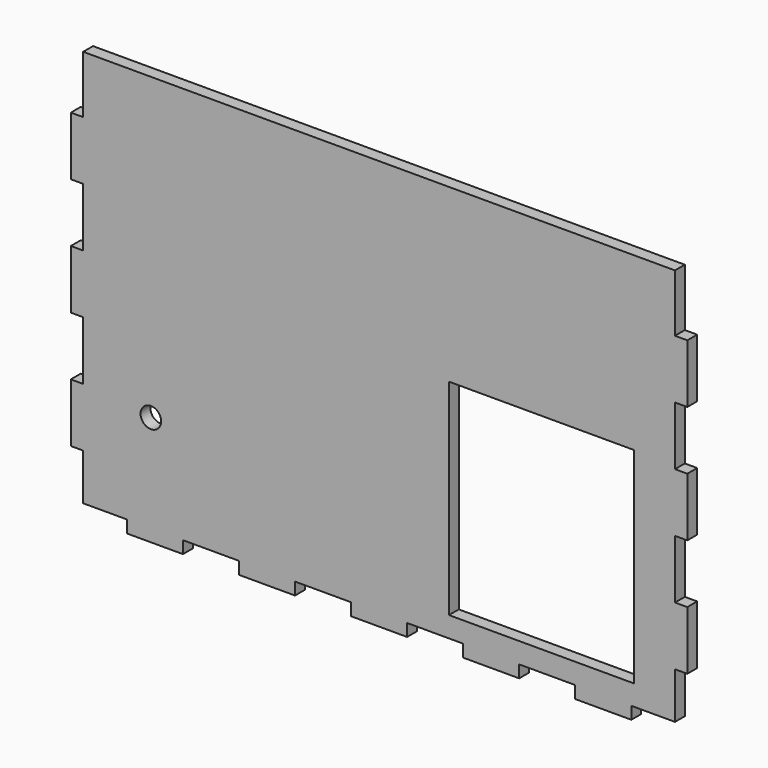
from build123d import *

# Parameters (mm, degrees)
F0_R     = 2.5
F0_W     = 45
F0_H     = 50
F1_DEPTH = 3


# Not quite as in the source:
# - ends of sketch curves that miss each other by under 0.0002 mm in the source are joined


with BuildPart() as f1:
    # F0 (on Front) → F1 (new body)
    with BuildSketch(Plane.XZ):
        Polygon((72.0000029802, 36.0006778365), (72.0000029802, 50), (-72.0000029802, 50), (-72.0000029802, 36.0006778365), (-75.0000029802, 36.0006778365), (-75.0000029802, 21.7149635505), (-72.0000029802, 21.7149635505), (-72.0000029802, 7.4292492645), (-75.0000029802, 7.4292492645), (-75.0000029802, -6.8564650215), (-72.0000029802, -6.8564650215), (-72.0000029802, -21.1421793075), (-75.0000029802, -21.1421793075), (-75.0000029802, -35.4278935935), (-72.0000029802, -35.4278935935), (-72.0000029802, -46.7136078775), (-61.363272724, -46.7136078775), (-61.363272724, -49.7136078775), (-47.726909088, -49.7136078775), (-47.726909088, -46.7136078775), (-34.090545452, -46.7136078775), (-34.090545452, -49.7136078775), (-20.454181816, -49.7136078775), (-20.454181816, -46.7136078775), (-6.81781818, -46.7136078775), (-6.81781818, -49.7136078775), (6.818545456, -49.7136078775), (6.818545456, -46.7136078775), (20.454909092, -46.7136078775), (20.454909092, -49.7136078775), (34.091272728, -49.7136078775), (34.091272728, -46.7136078775), (47.727636364, -46.7136078775), (47.727636364, -49.7136078775), (61.364, -49.7136078775), (61.364, -46.7136078775), (72.0000029802, -46.7136078775), (72.0000029802, -35.4278935935), (75.0000029802, -35.4278935935), (75.0000029802, -21.1421793075), (72.0000029802, -21.1421793075), (72.0000029802, -6.8564650215), (75.0000029802, -6.8564650215), (75.0000029802, 7.4292492645), (72.0000029802, 7.4292492645), (72.0000029802, 21.7149635505), (75.0000029802, 21.7149635505), (75.0000029802, 36.0006778365), align=None)
        with Locations((-55.5279403925, -22.991552949)):
            Circle(F0_R, mode=Mode.SUBTRACT)
        with Locations((39.5000029802, -16.7136078775)):
            Rectangle(F0_W, F0_H, mode=Mode.SUBTRACT)
    extrude(amount=F1_DEPTH)


solid = f1.part
